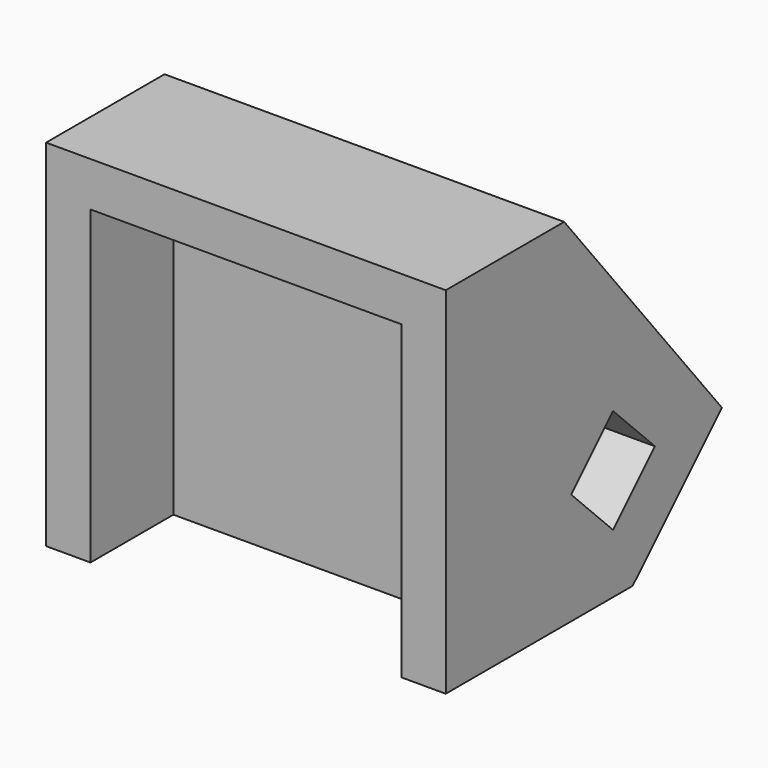
from build123d import *

# Parameters (mm, degrees)
F0_W          = 10.5
F0_H          = 10.5
F1_DEPTH      = 1.5
F3_DEPTH      = 5
F5_DEPTH      = 6.75
F5_DEPTH_BACK = 6.75


# Not quite as in the source:
# - an extrude ends at something that could not be found from the text; its depth is read off the source's solid


with BuildPart() as f1:
    # F0 (on Front) → F1 (new body)
    with BuildSketch(Plane.XZ):
        Rectangle(F0_W, F0_H)
    extrude(amount=F1_DEPTH)

    # F2 (on face) → F3 (join)
    with BuildSketch(Plane(origin=(0, 0, 0), x_dir=(-1, 0, 0), z_dir=(0, 1, 0))):
        Polygon((-6.75, -5.25), (-5.25, -5.25), (-5.25, 5.25), (5.25, 5.25), (5.25, -5.25), (6.75, -5.25), (6.75, 6.75), (-6.75, 6.75), align=None)
    extrude(amount=-F3_DEPTH)

    # F4 (on Right) → F5 (join, two sides)
    with BuildSketch(Plane.YZ) as f5_sk:
        Polygon((0, 6.75), (0, -5.25), (2.8927646712, -5.25), (6.6605316242, -1.482233047), align=None)
        Polygon((2.0643375465, -3.25), (0.2965705935, -1.482233047), (2.0643375465, 0.2855339059), (3.8321044994, -1.482233047), align=None, mode=Mode.SUBTRACT)
    extrude(amount=F5_DEPTH)
    extrude(f5_sk.sketch, amount=-F5_DEPTH_BACK)


solid = f1.part
